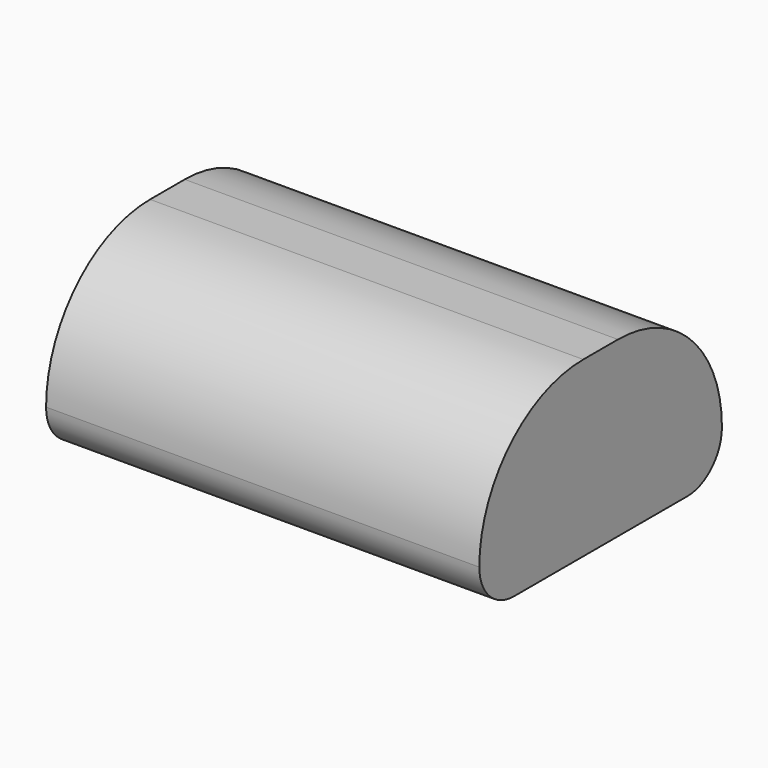
from build123d import *

# Parameters (mm, degrees)
F0_W     = 1000
F0_H     = 700
F1_DEPTH = 400
F2_R     = 300
F3_R     = 99.99999


# Not quite as in the source:
# - a fillet or chamfer is up to 0.001 mm smaller than in the source, because OpenCascade refuses the exact size


with BuildPart() as f1:
    # F0 (on Top) → F1 (new body)
    with BuildSketch(Plane.XY):
        Rectangle(F0_W, F0_H)
    extrude(amount=F1_DEPTH)

    # F2
    f2_edges = [f1.edges().sort_by_distance(p)[0] for p in [
        (0, -350, 400),
        (0, 350, 400),
    ]]
    fillet(f2_edges, radius=F2_R)

    # F3 (radius 100 in the source; OpenCascade refuses exactly that, so slightly less here)
    f3_edges = [f1.edges().sort_by_distance(p)[0] for p in [
        (0, 350, 0),
        (0, -350, 0),
    ]]
    fillet(f3_edges, radius=F3_R)


solid = f1.part
